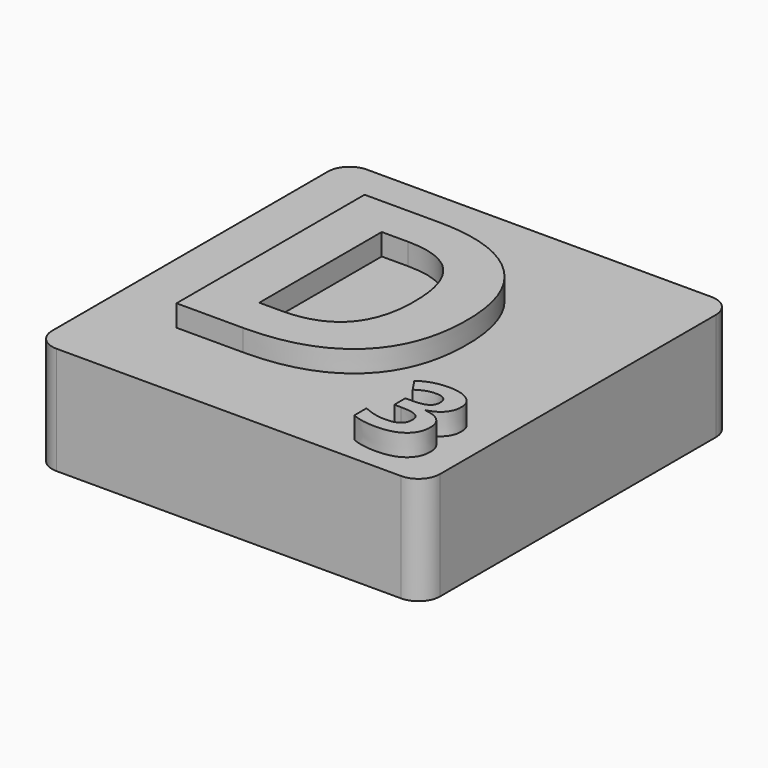
from build123d import *

# Parameters (mm, degrees)
F0_W           = 18
F0_H           = 18
F1_DEPTH       = 5
F2_W           = 16
F2_H           = 16
F3_DEPTH       = 3
F4_TEXT_SIZE   = 15.2777777778
F4_TEXT_SIZE_2 = 5.5555555556
F5_DEPTH       = 1
F6_R           = 1


# Not quite as in the source:
# - Text() gives the source's letters only with a copy of the font that has no kerning and outlines rounded to 1/6400 em; it was checked with that copy


with BuildPart() as f1:
    # F0 (on Top) → F1 (new body)
    with BuildSketch(Plane.XY):
        with Locations((5.0695089158, -1.7574313941)):
            Rectangle(F0_W, F0_H)
    extrude(amount=F1_DEPTH)

    # F2 (on Top) → F3 (cut)
    with BuildSketch(Plane.XY):
        with Locations((5.0695089158, -1.7574313941)):
            Rectangle(F2_W, F2_H)
    extrude(amount=F3_DEPTH, mode=Mode.SUBTRACT)

    # F4 (on face) → F5 (join)
    with BuildSketch(Plane.XY.offset(5)):
        with Locations((-1.9304910842, -6.7574313941)):
            Text('D', F4_TEXT_SIZE, font='Open Sans', font_style=FontStyle.BOLD, text_align=(TextAlign.LEFT, TextAlign.BOTTOM))
        with Locations((9.752668638, -9.7574313941)):
            Text('3', F4_TEXT_SIZE_2, font='Open Sans', font_style=FontStyle.BOLD, text_align=(TextAlign.LEFT, TextAlign.BOTTOM))
    extrude(amount=F5_DEPTH)

    # F6
    f6_edges = [f1.edges().sort_by_distance(p)[0] for p in [
        (14.069509, 7.242569, 2.5),
        (14.069509, -10.757431, 2.5),
        (-3.930491, -10.757431, 2.5),
        (-3.930491, 7.242569, 2.5),
        (13.069509, -9.757431, 1.5),
        (-2.930491, -9.757431, 1.5),
        (-2.930491, 6.242569, 1.5),
        (13.069509, 6.242569, 1.5),
    ]]
    fillet(f6_edges, radius=F6_R)


solid = f1.part
